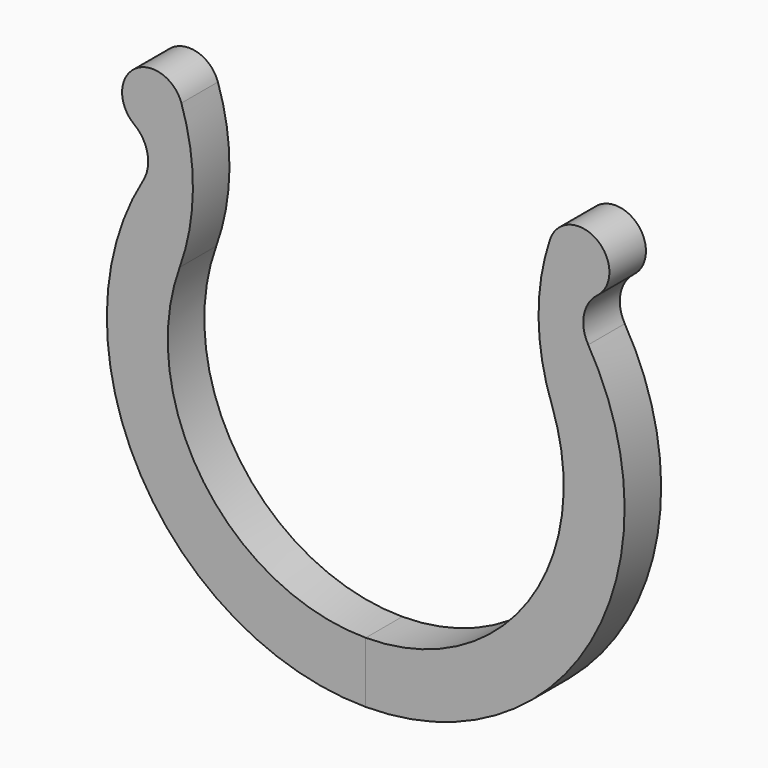
from build123d import *
from build123d import SkipClean  # not in build123d's __all__

# Parameters (mm, degrees)
F1_DEPTH = 0.9


with BuildPart() as f1:
    # F0 (on Front) → F1 (new body)
    with BuildSketch(Plane.XZ):
        with BuildLine():
            ThreePointArc((-3.6648012211, 1.333878559), (-3.4047554287, 2.7601313999), (-3.6315648982, 4.1920456588))
            ThreePointArc((-3.6315648982, 4.1920456588), (-4.5505468427, 4.4869465177), (-4.562494352, 3.5218809304))
            ThreePointArc((-4.562494352, 3.5218809304), (-4.2983800559, 3.0982301484), (-4.3837176879, 2.6063421173))
            ThreePointArc((-4.3837176879, 2.6063421173), (-4.4329642903, -2.5216715886), (0, -5.1))
            Line((0, -5.1), (0, -3.9))
            ThreePointArc((0, -3.9), (-3.1946929727, -2.2369481018), (-3.6648012211, 1.333878559))
        make_face()
    extrude(amount=F1_DEPTH)

    # F2: F1 across plane


with BuildPart() as f1_1:
    add(f1.part, clean=False)
    with SkipClean():  # cleaning this boolean's faces spoils the solid; the shape is the same uncleaned
        add(f1.part.mirror(Plane.YZ), clean=False)


solid = f1_1.part
